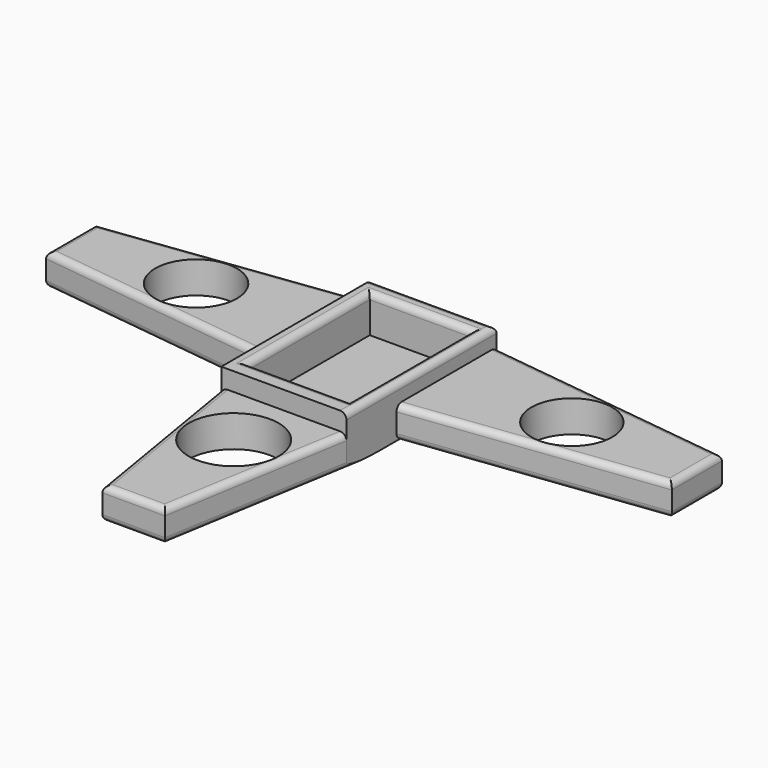
from build123d import *

# Parameters (mm, degrees)
F0_W           = 100
F0_H           = 100
F1_DEPTH       = 40
F2_DEPTH       = 10
F3_DEPTH       = 10
F0_H_2         = 50
F4_DEPTH       = 25.4
F5_DEPTH       = 40
F6_R           = 32.6138389822
F6_R_2         = 35.8864920554
F6_R_3         = 32.2738018283
F7_DEPTH       = 51.308
F8_W           = 80
F8_H           = 130
F9_DEPTH       = 40
F10_W          = 81.0131505132
F10_H          = 121.7317990959
F11_DEPTH      = 30
F12_T1_DEPTH   = 75.4
F12_T3_DEPTH   = 175.4
F12_T5_DEPTH   = 121.7317990959
F12_T7_DEPTH   = 81.0131505132
F12_T9_DEPTH   = 125.4
F12_T11_DEPTH  = 74.6412090302
F12_T13_DEPTH  = 75.4
F12_T15_DEPTH  = 202.8690632575
F12_T17_DEPTH  = 202.8690632575
F12_T19_DEPTH  = 277.851965803
F12_T21_DEPTH  = 227
F12_T23_DEPTH  = 277.7564437075
F12_T28_DEPTH  = 277.7564437075
F12_T33_DEPTH  = 226.9564437075
F12_T38_DEPTH  = 277.851965803
F12_T43_DEPTH  = 226.9564437075
F12_T48_DEPTH  = 202.8690632575
F12_T53_DEPTH  = 202.8690632575
F12_T58_DEPTH  = 226.9564437075
F12_T63_DEPTH  = 226.9564437075
F12_T69_DEPTH  = 93.7131505132
F12_T74_DEPTH  = 134.4317990959
F12_T81_DEPTH  = 93.7131505132
F12_T86_DEPTH  = 134.4317990959
F12_T93_DEPTH  = 93.7131505132
F12_T98_DEPTH  = 134.4317990959
F12_T105_DEPTH = 134.4317990959
F12_T109_DEPTH = 93.7131505132


# Not quite as in the source:
# - a fillet or chamfer that OpenCascade refuses, or shapes differently, is made with other operations: its cross-section is extruded or revolved along the edge and cut away or added


with BuildPart() as f1:
    # F0 (on Top) → F1 (new body)
    with BuildSketch(Plane.XY):
        Rectangle(F0_W, F0_H)
    extrude(amount=F1_DEPTH)

    # F0 (on Top) → F2 (join)
    with BuildSketch(Plane.XY):
        Polygon((250, 25), (50, 50), (50, -50), (250, -25), align=None)
    extrude(amount=F2_DEPTH)

    # F0 (on Top) → F3 (join)
    with BuildSketch(Plane.XY):
        Polygon((-50, -50), (-50, 50), (-250, 24.2412090302), (-250, -25), align=None)
    extrude(amount=F3_DEPTH)

    # F0 (on Top) → F4 (join)
    with BuildSketch(Plane.XY):
        Rectangle(F0_W, F0_H)
        Polygon((250, 25), (50, 50), (50, -50), (250, -25), align=None)
        Polygon((-50, -50), (-50, 50), (-250, 24.2412090302), (-250, -25), align=None)
        with Locations((0, -75)):
            Rectangle(F0_W, F0_H_2)
        Polygon((25, -250), (50, -100), (-50, -100), (-25, -250), align=None)
    extrude(amount=F4_DEPTH)

    # F0 (on Top) → F5 (join)
    with BuildSketch(Plane.XY):
        with Locations((0, -75)):
            Rectangle(F0_W, F0_H_2)
    extrude(amount=F5_DEPTH)

    # F6 (on face) → F7 (cut)
    with BuildSketch(Plane.XY.offset(25.4)):
        with Locations((-150, -0.1896977425)):
            Circle(F6_R)
        with Locations((0.1525683302, -150.3578271792)):
            Circle(F6_R_2)
        with Locations((150.1342882352, -0.0758587057)):
            Circle(F6_R_3)
    extrude(amount=-F7_DEPTH, mode=Mode.SUBTRACT)

    # F8 (on face) → F9 (join)
    with BuildSketch(Plane.XY.offset(40)):
        with Locations((0, -25)):
            Rectangle(F8_W, F8_H)
    extrude(amount=-F9_DEPTH)

    # F10 (on face) → F11 (cut)
    with BuildSketch(Plane.XY.offset(40)):
        with Locations((0.2870373428, -24.8173717409)):
            Rectangle(F10_W, F10_H)
    extrude(amount=-F11_DEPTH, mode=Mode.SUBTRACT)

    # F12: fillet of radius 5.08 on 25 edges, made by hand

    # F12_s2 → F12_t1 (cut)
    with BuildSketch(Plane.XZ.offset(-37.7)):
        with BuildLine():
            ThreePointArc((250, 20.32), (248.5121024484, 23.9121024484), (244.92, 25.4))
            Line((244.92, 25.4), (250, 25.4))
            Line((250, 25.4), (250, 20.32))
        make_face()
        with BuildLine():
            ThreePointArc((244.92, 0), (248.5121024484, 1.4878975516), (250, 5.08))
            Line((250, 5.08), (250, 0))
            Line((250, 0), (244.92, 0))
        make_face()
    extrude(amount=F12_T1_DEPTH, mode=Mode.SUBTRACT)

    # F12_s4 → F12_t3 (cut)
    with BuildSketch(Plane.XZ.offset(-62.7)):
        with BuildLine():
            ThreePointArc((50, 34.92), (48.5121024484, 38.5121024484), (44.92, 40))
            Line((44.92, 40), (50, 40))
            Line((50, 40), (50, 34.92))
        make_face()
    extrude(amount=F12_T3_DEPTH, mode=Mode.SUBTRACT)

    # F12_s6 → F12_t5 (cut)
    with BuildSketch(Plane.XZ.offset(-36.048527807)):
        with BuildLine():
            ThreePointArc((45.8736125994, 40), (42.2815101509, 38.5121024484), (40.7936125994, 34.92))
            Line((40.7936125994, 34.92), (40.7936125994, 40))
            Line((40.7936125994, 40), (45.8736125994, 40))
        make_face()
        with BuildLine():
            ThreePointArc((-45.2995379138, 40), (-41.7074354654, 38.5121024484), (-40.2195379138, 34.92))
            Line((-40.2195379138, 34.92), (-40.2195379138, 40))
            Line((-40.2195379138, 40), (-45.2995379138, 40))
        make_face()
    extrude(amount=F12_T5_DEPTH, mode=Mode.SUBTRACT)

    # F12_s8 → F12_t7 (cut)
    with BuildSketch(Plane.YZ.offset(-40.2195379138)):
        with BuildLine():
            ThreePointArc((41.128527807, 40), (37.5364253586, 38.5121024484), (36.048527807, 34.92))
            Line((36.048527807, 34.92), (36.048527807, 40))
            Line((36.048527807, 40), (41.128527807, 40))
        make_face()
        with BuildLine():
            ThreePointArc((-90.7632712889, 40), (-87.1711688404, 38.5121024484), (-85.6832712889, 34.92))
            Line((-85.6832712889, 34.92), (-85.6832712889, 40))
            Line((-85.6832712889, 40), (-90.7632712889, 40))
        make_face()
    extrude(amount=F12_T7_DEPTH, mode=Mode.SUBTRACT)

    # F12_s10 → F12_t9 (cut)
    with BuildSketch(Plane.YZ.offset(-62.7)):
        with BuildLine():
            ThreePointArc((50, 34.92), (48.5121024484, 38.5121024484), (44.92, 40))
            Line((44.92, 40), (50, 40))
            Line((50, 40), (50, 34.92))
        make_face()
    extrude(amount=F12_T9_DEPTH, mode=Mode.SUBTRACT)

    # F12_s12 → F12_t11 (cut)
    with BuildSketch(Plane.XZ.offset(-36.9412090302)):
        with BuildLine():
            ThreePointArc((-250, 20.32), (-248.5121024484, 23.9121024484), (-244.92, 25.4))
            Line((-244.92, 25.4), (-250, 25.4))
            Line((-250, 25.4), (-250, 20.32))
        make_face()
        with BuildLine():
            ThreePointArc((-244.92, 0), (-248.5121024484, 1.4878975516), (-250, 5.08))
            Line((-250, 5.08), (-250, 0))
            Line((-250, 0), (-244.92, 0))
        make_face()
    extrude(amount=F12_T11_DEPTH, mode=Mode.SUBTRACT)

    # F12_s14 → F12_t13 (cut)
    with BuildSketch(Plane.YZ.offset(-37.7)):
        with BuildLine():
            ThreePointArc((-250, 20.32), (-248.5121024484, 23.9121024484), (-244.92, 25.4))
            Line((-244.92, 25.4), (-250, 25.4))
            Line((-250, 25.4), (-250, 20.32))
        make_face()
        with BuildLine():
            ThreePointArc((-244.92, 0), (-248.5121024484, 1.4878975516), (-250, 5.08))
            Line((-250, 5.08), (-250, 0))
            Line((-250, 0), (-244.92, 0))
        make_face()
    extrude(amount=F12_T13_DEPTH, mode=Mode.SUBTRACT)

    # F12_s16 → F12_t15 (cut)
    with BuildSketch(Plane(origin=(-41.9527320036, -251.7163920219, 0), x_dir=(0, 0, 1), z_dir=(0.1643989873, 0.9863939238, 0))):
        with BuildLine():
            ThreePointArc((0, 60.6795949221), (1.4878975516, 64.2716973706), (5.08, 65.7595949221))
            Line((5.08, 65.7595949221), (0, 65.7595949221))
            Line((0, 65.7595949221), (0, 60.6795949221))
        make_face()
    extrude(amount=F12_T15_DEPTH, mode=Mode.SUBTRACT)

    # F12_s18 → F12_t17 (cut)
    with BuildSketch(Plane(origin=(8.6012634485, -51.6075806912, 0), x_dir=(0, 0, 1), z_dir=(0.1643989873, -0.9863939238, 0))):
        with BuildLine():
            ThreePointArc((0, 60.6795949221), (1.4878975516, 64.2716973706), (5.08, 65.7595949221))
            Line((5.08, 65.7595949221), (0, 65.7595949221))
            Line((0, 65.7595949221), (0, 60.6795949221))
        make_face()
    extrude(amount=F12_T17_DEPTH, mode=Mode.SUBTRACT)

    # F12_s20 → F12_t19 (cut)
    with BuildSketch(Plane(origin=(20.1302781895, 2.5926581402, 0), x_dir=(0, 0, 1), z_dir=(-0.9918078369, -0.1277388538, 0))):
        with BuildLine():
            ThreePointArc((0, 50.8973345305), (1.4878975516, 54.4894369789), (5.08, 55.9773345305))
            Line((5.08, 55.9773345305), (0, 55.9773345305))
            Line((0, 55.9773345305), (0, 50.8973345305))
        make_face()
    extrude(amount=F12_T19_DEPTH, mode=Mode.SUBTRACT)

    # F12_s22 → F12_t21 (cut)
    with BuildSketch(Plane.YZ.offset(-113.5)):
        with BuildLine():
            ThreePointArc((50, 5.08), (48.5121024484, 1.4878975516), (44.92, 0))
            Line((44.92, 0), (50, 0))
            Line((50, 0), (50, 5.08))
        make_face()
    extrude(amount=F12_T21_DEPTH, mode=Mode.SUBTRACT)

    # F12_s24 → F12_t23 (cut)
    with BuildSketch(Plane(origin=(255.6788521112, -31.9598565139, 0), x_dir=(0, 0, 1), z_dir=(-0.9922778767, 0.1240347346, 0))):
        with BuildLine():
            ThreePointArc((0, 50.7356305651), (1.4878975516, 54.3277330136), (5.08, 55.8156305651))
            Line((5.08, 55.8156305651), (0, 55.8156305651))
            Line((0, 55.8156305651), (0, 50.7356305651))
        make_face()
    extrude(amount=F12_T23_DEPTH, mode=Mode.SUBTRACT)


with BuildPart() as f12_tool26:
    # F12_s27 → F12_t28 (new body)
    with BuildSketch(Plane(origin=(255.6788521112, -31.9598565139, 0), x_dir=(0, 0, 1), z_dir=(-0.9922778767, 0.1240347346, 0))):
        with BuildLine():
            ThreePointArc((20.32, 55.8156305651), (23.9121024484, 54.3277330136), (25.4, 50.7356305651))
            Line((25.4, 50.7356305651), (25.4, 55.8156305651))
            Line((25.4, 55.8156305651), (20.32, 55.8156305651))
        make_face()
    extrude(amount=F12_T28_DEPTH)

    split(bisect_by=Plane.YZ.offset(50), keep=Keep.TOP)


with BuildPart() as f1_1:
    add(f1.part)

    # F12_t25: cut F12_tool26
    add(f12_tool26.part, mode=Mode.SUBTRACT)


with BuildPart() as f12_tool31:
    # F12_s32 → F12_t33 (new body)
    with BuildSketch(Plane(origin=(30.4749940427, 3.8093742553, 0), x_dir=(0, 0, 1), z_dir=(0.9922778767, 0.1240347346, 0))):
        with BuildLine():
            ThreePointArc((20.32, 55.8156305651), (23.9121024484, 54.3277330136), (25.4, 50.7356305651))
            Line((25.4, 50.7356305651), (25.4, 55.8156305651))
            Line((25.4, 55.8156305651), (20.32, 55.8156305651))
        make_face()
    extrude(amount=F12_T33_DEPTH)

    split(bisect_by=Plane.YZ.offset(50), keep=Keep.TOP)


with BuildPart() as f1_2:
    add(f1_1.part)

    # F12_t30: cut F12_tool31
    add(f12_tool31.part, mode=Mode.SUBTRACT)


with BuildPart() as f12_tool36:
    # F12_s37 → F12_t38 (new body)
    with BuildSketch(Plane(origin=(20.1302781895, 2.5926581402, 0), x_dir=(0, 0, 1), z_dir=(-0.9918078369, -0.1277388538, 0))):
        with BuildLine():
            ThreePointArc((20.32, 55.9773345305), (23.9121024484, 54.4894369789), (25.4, 50.8973345305))
            Line((25.4, 50.8973345305), (25.4, 55.9773345305))
            Line((25.4, 55.9773345305), (20.32, 55.9773345305))
        make_face()
    extrude(amount=F12_T38_DEPTH)

    split(bisect_by=Plane.YZ.offset(-50), keep=Keep.BOTTOM)


with BuildPart() as f1_3:
    add(f1_2.part)

    # F12_t35: cut F12_tool36
    add(f12_tool36.part, mode=Mode.SUBTRACT)


with BuildPart() as f12_tool41:
    # F12_s42 → F12_t43 (new body)
    with BuildSketch(Plane(origin=(-255.6788521112, 31.9598565139, 0), x_dir=(0, 0, 1), z_dir=(0.9922778767, -0.1240347346, 0))):
        with BuildLine():
            ThreePointArc((20.32, 55.8156305651), (23.9121024484, 54.3277330136), (25.4, 50.7356305651))
            Line((25.4, 50.7356305651), (25.4, 55.8156305651))
            Line((25.4, 55.8156305651), (20.32, 55.8156305651))
        make_face()
    extrude(amount=F12_T43_DEPTH)

    split(bisect_by=Plane.YZ.offset(-50), keep=Keep.BOTTOM)


with BuildPart() as f1_4:
    add(f1_3.part)

    # F12_t40: cut F12_tool41
    add(f12_tool41.part, mode=Mode.SUBTRACT)


with BuildPart() as f12_tool46:
    # F12_s47 → F12_t48 (new body)
    with BuildSketch(Plane(origin=(8.6012634485, -51.6075806912, 0), x_dir=(0, 0, 1), z_dir=(0.1643989873, -0.9863939238, 0))):
        with BuildLine():
            ThreePointArc((20.32, 65.7595949221), (23.9121024484, 64.2716973706), (25.4, 60.6795949221))
            Line((25.4, 60.6795949221), (25.4, 65.7595949221))
            Line((25.4, 65.7595949221), (20.32, 65.7595949221))
        make_face()
    extrude(amount=F12_T48_DEPTH)

    split(bisect_by=Plane.XZ.offset(100), keep=Keep.TOP)


with BuildPart() as f1_5:
    add(f1_4.part)

    # F12_t45: cut F12_tool46
    add(f12_tool46.part, mode=Mode.SUBTRACT)


with BuildPart() as f12_tool51:
    # F12_s52 → F12_t53 (new body)
    with BuildSketch(Plane(origin=(-41.9527320036, -251.7163920219, 0), x_dir=(0, 0, 1), z_dir=(0.1643989873, 0.9863939238, 0))):
        with BuildLine():
            ThreePointArc((20.32, 65.7595949221), (23.9121024484, 64.2716973706), (25.4, 60.6795949221))
            Line((25.4, 60.6795949221), (25.4, 65.7595949221))
            Line((25.4, 65.7595949221), (20.32, 65.7595949221))
        make_face()
    extrude(amount=F12_T53_DEPTH)

    split(bisect_by=Plane.XZ.offset(100), keep=Keep.TOP)


with BuildPart() as f1_6:
    add(f1_5.part)

    # F12_t50: cut F12_tool51
    add(f12_tool51.part, mode=Mode.SUBTRACT)


with BuildPart() as f12_tool56:
    # F12_s57 → F12_t58 (new body)
    with BuildSketch(Plane(origin=(-255.6788521112, 31.9598565139, 0), x_dir=(0, 0, 1), z_dir=(0.9922778767, -0.1240347346, 0))):
        with BuildLine():
            ThreePointArc((0, 50.7356305651), (1.4878975516, 54.3277330136), (5.08, 55.8156305651))
            Line((5.08, 55.8156305651), (0, 55.8156305651))
            Line((0, 55.8156305651), (0, 50.7356305651))
        make_face()
    extrude(amount=F12_T58_DEPTH)

    split(bisect_by=Plane.YZ.offset(-50), keep=Keep.BOTTOM)


with BuildPart() as f1_7:
    add(f1_6.part)

    # F12_t55: cut F12_tool56
    add(f12_tool56.part, mode=Mode.SUBTRACT)


with BuildPart() as f12_tool61:
    # F12_s62 → F12_t63 (new body)
    with BuildSketch(Plane(origin=(30.4749940427, 3.8093742553, 0), x_dir=(0, 0, 1), z_dir=(0.9922778767, 0.1240347346, 0))):
        with BuildLine():
            ThreePointArc((0, 50.7356305651), (1.4878975516, 54.3277330136), (5.08, 55.8156305651))
            Line((5.08, 55.8156305651), (0, 55.8156305651))
            Line((0, 55.8156305651), (0, 50.7356305651))
        make_face()
    extrude(amount=F12_T63_DEPTH)

    split(bisect_by=Plane.YZ.offset(50), keep=Keep.TOP)


with BuildPart() as f1_8:
    add(f1_7.part)

    # F12_t60: cut F12_tool61
    add(f12_tool61.part, mode=Mode.SUBTRACT)


with BuildPart() as f12_tool67:
    # F12_s68 → F12_t69 (new body)
    with BuildSketch(Plane.YZ.offset(-40.2195379138)):
        with BuildLine():
            ThreePointArc((-90.7632712889, 40), (-87.1711688404, 38.5121024484), (-85.6832712889, 34.92))
            Line((-85.6832712889, 34.92), (-85.6832712889, 40))
            Line((-85.6832712889, 40), (-90.7632712889, 40))
        make_face()
    extrude(amount=F12_T69_DEPTH)

    split(bisect_by=Plane.YZ.offset(50), keep=Keep.BOTTOM)

    split(bisect_by=Plane.YZ.offset(40.7936125994), keep=Keep.TOP)


with BuildPart() as f12_tool72:
    # F12_s73 → F12_t74 (new body)
    with BuildSketch(Plane.XZ.offset(98.3832712889)):
        with BuildLine():
            ThreePointArc((45.8736125994, 40), (42.2815101509, 38.5121024484), (40.7936125994, 34.92))
            Line((40.7936125994, 34.92), (40.7936125994, 40))
            Line((40.7936125994, 40), (45.8736125994, 40))
        make_face()
    extrude(amount=-F12_T74_DEPTH)

    split(bisect_by=Plane.XZ.offset(85.6832712889), keep=Keep.TOP)


with BuildPart() as f12_tool67_1:
    add(f12_tool67.part)

    # F12_t76: intersect F12_tool72
    add(f12_tool72.part, mode=Mode.INTERSECT)


with BuildPart() as f1_9:
    add(f1_8.part)

    # F12_t65: cut F12_tool67
    add(f12_tool67_1.part, mode=Mode.SUBTRACT)


with BuildPart() as f12_tool79:
    # F12_s80 → F12_t81 (new body)
    with BuildSketch(Plane.YZ.offset(53.4936125994)):
        with BuildLine():
            ThreePointArc((41.128527807, 40), (37.5364253586, 38.5121024484), (36.048527807, 34.92))
            Line((36.048527807, 34.92), (36.048527807, 40))
            Line((36.048527807, 40), (41.128527807, 40))
        make_face()
    extrude(amount=-F12_T81_DEPTH)

    split(bisect_by=Plane.YZ.offset(50), keep=Keep.BOTTOM)

    split(bisect_by=Plane.YZ.offset(40.7936125994), keep=Keep.TOP)


with BuildPart() as f12_tool84:
    # F12_s85 → F12_t86 (new body)
    with BuildSketch(Plane.XZ.offset(85.6832712889)):
        with BuildLine():
            ThreePointArc((45.8736125994, 40), (42.2815101509, 38.5121024484), (40.7936125994, 34.92))
            Line((40.7936125994, 34.92), (40.7936125994, 40))
            Line((40.7936125994, 40), (45.8736125994, 40))
        make_face()
    extrude(amount=-F12_T86_DEPTH)

    split(bisect_by=Plane.XZ.offset(-36.048527807), keep=Keep.BOTTOM)


with BuildPart() as f12_tool79_1:
    add(f12_tool79.part)

    # F12_t88: intersect F12_tool84
    add(f12_tool84.part, mode=Mode.INTERSECT)


with BuildPart() as f1_10:
    add(f1_9.part)

    # F12_t77: cut F12_tool79
    add(f12_tool79_1.part, mode=Mode.SUBTRACT)


with BuildPart() as f12_tool91:
    # F12_s92 → F12_t93 (new body)
    with BuildSketch(Plane.YZ.offset(40.7936125994)):
        with BuildLine():
            ThreePointArc((41.128527807, 40), (37.5364253586, 38.5121024484), (36.048527807, 34.92))
            Line((36.048527807, 34.92), (36.048527807, 40))
            Line((36.048527807, 40), (41.128527807, 40))
        make_face()
    extrude(amount=-F12_T93_DEPTH)

    split(bisect_by=Plane.YZ.offset(-50), keep=Keep.TOP)

    split(bisect_by=Plane.YZ.offset(-40.2195379138), keep=Keep.BOTTOM)


with BuildPart() as f12_tool96:
    # F12_s97 → F12_t98 (new body)
    with BuildSketch(Plane.XZ.offset(-48.748527807)):
        with BuildLine():
            ThreePointArc((-45.2995379138, 40), (-41.7074354654, 38.5121024484), (-40.2195379138, 34.92))
            Line((-40.2195379138, 34.92), (-40.2195379138, 40))
            Line((-40.2195379138, 40), (-45.2995379138, 40))
        make_face()
    extrude(amount=F12_T98_DEPTH)

    split(bisect_by=Plane.XZ.offset(-36.048527807), keep=Keep.BOTTOM)


with BuildPart() as f12_tool91_1:
    add(f12_tool91.part)

    # F12_t100: intersect F12_tool96
    add(f12_tool96.part, mode=Mode.INTERSECT)


with BuildPart() as f1_11:
    add(f1_10.part)

    # F12_t89: cut F12_tool91
    add(f12_tool91_1.part, mode=Mode.SUBTRACT)


with BuildPart() as f12_tool103:
    # F12_s104 → F12_t105 (new body)
    with BuildSketch(Plane.XZ.offset(-36.048527807)):
        with BuildLine():
            ThreePointArc((-45.2995379138, 40), (-41.7074354654, 38.5121024484), (-40.2195379138, 34.92))
            Line((-40.2195379138, 34.92), (-40.2195379138, 40))
            Line((-40.2195379138, 40), (-45.2995379138, 40))
        make_face()
    extrude(amount=F12_T105_DEPTH)

    split(bisect_by=Plane.XZ.offset(85.6832712889), keep=Keep.TOP)


with BuildPart() as f12_tool107:
    # F12_s108 → F12_t109 (new body)
    with BuildSketch(Plane.YZ.offset(-52.9195379138)):
        with BuildLine():
            ThreePointArc((-90.7632712889, 40), (-87.1711688404, 38.5121024484), (-85.6832712889, 34.92))
            Line((-85.6832712889, 34.92), (-85.6832712889, 40))
            Line((-85.6832712889, 40), (-90.7632712889, 40))
        make_face()
    extrude(amount=F12_T109_DEPTH)

    split(bisect_by=Plane.YZ.offset(-50), keep=Keep.TOP)

    split(bisect_by=Plane.YZ.offset(-40.2195379138), keep=Keep.BOTTOM)


with BuildPart() as f12_tool103_1:
    add(f12_tool103.part)

    # F12_t112: intersect F12_tool107
    add(f12_tool107.part, mode=Mode.INTERSECT)


with BuildPart() as f1_12:
    add(f1_11.part)

    # F12_t101: cut F12_tool103
    add(f12_tool103_1.part, mode=Mode.SUBTRACT)


solid = f1_12.part
